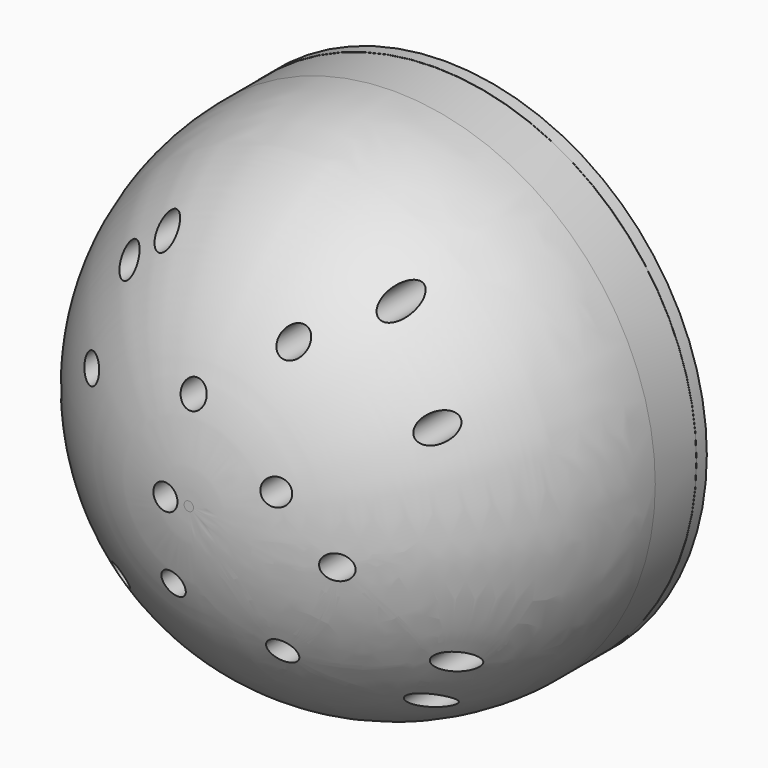
from build123d import *

# Parameters (mm, degrees)
F0_R     = 20.3669394185
F0_R_2   = 1
F1_DEPTH = 25
F3_R     = 20.3845916769
F4_DEPTH = 1


# Not quite as in the source:
# - a fillet or chamfer that OpenCascade refuses, or shapes differently, is made with other operations: its cross-section is extruded or revolved along the edge and cut away or added


with BuildPart() as f1:
    # F0 (on Front) → F1 (new body)
    with BuildSketch(Plane.XZ):
        Circle(F0_R)
        with Locations((-11.1758968817, -14.00543161)):
            Circle(F0_R_2, mode=Mode.SUBTRACT)
        with Locations((-1.890650721, -16.7809611674)):
            Circle(F0_R_2, mode=Mode.SUBTRACT)
        with Locations((-8.9275289642, -9.4687726276)):
            Circle(F0_R_2, mode=Mode.SUBTRACT)
        with Locations((-2.0294538699, -6.3785142265)):
            Circle(F0_R_2, mode=Mode.SUBTRACT)
        with Locations((10.9048346058, -13.7971816584)):
            Circle(F0_R_2, mode=Mode.SUBTRACT)
        with Locations((4.980258228, -9.4945097982)):
            Circle(F0_R_2, mode=Mode.SUBTRACT)
        with Locations((9.6366257886, -2.0369203499)):
            Circle(F0_R_2, mode=Mode.SUBTRACT)
        with Locations((13.7883136049, -9.743324481)):
            Circle(F0_R_2, mode=Mode.SUBTRACT)
        with Locations((-16.2434000522, 0)):
            Circle(F0_R_2, mode=Mode.SUBTRACT)
        with Locations((-10.1784534926, 4.8293601592)):
            Circle(F0_R_2, mode=Mode.SUBTRACT)
        with Locations((-1.890650721, 0)):
            Circle(F0_R_2, mode=Mode.SUBTRACT)
        with Locations((-0.5644357263, 7.0376366864)):
            Circle(F0_R_2, mode=Mode.SUBTRACT)
        with Locations((-9.5657140447, 11.2727972235)):
            Circle(F0_R_2, mode=Mode.SUBTRACT)
        with Locations((-7.252750682, 13.6961765275)):
            Circle(F0_R_2, mode=Mode.SUBTRACT)
        with Locations((6.0194581747, 2.5240709074)):
            Circle(F0_R_2, mode=Mode.SUBTRACT)
        with Locations((13.7883136049, 7.0376366864)):
            Circle(F0_R_2, mode=Mode.SUBTRACT)
        with Locations((4.980258228, 11.2727972235)):
            Circle(F0_R_2, mode=Mode.SUBTRACT)
        with Locations((9.6366257886, 13.6961765275)):
            Circle(F0_R_2, mode=Mode.SUBTRACT)
    extrude(amount=F1_DEPTH)

    # F2: fillet of radius 20 on 1 edges, made by hand

    # F2_s1 → F2_t2 (revolve, cut)
    with BuildSketch(Plane.XY):
        with BuildLine():
            ThreePointArc((20.3669394185, -5), (14.5090750423, -19.1421356237), (0.3669394185, -25))
            Line((0.3669394185, -25), (20.3669394185, -25))
            Line((20.3669394185, -25), (20.3669394185, -5))
        make_face()
    revolve(axis=Axis((0, -25, 0), (0, -1, 0)), mode=Mode.SUBTRACT)

    # F3 (on Front) → F4 (join)
    with BuildSketch(Plane.XZ):
        Circle(F3_R)
    extrude(amount=F4_DEPTH)


solid = f1.part
